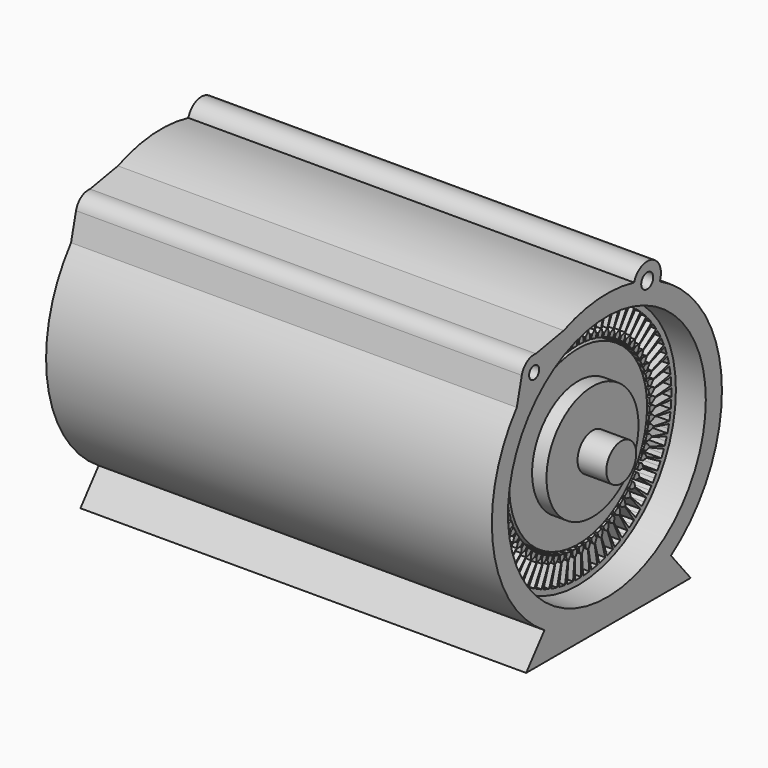
from build123d import *

# Parameters (mm, degrees)
F0_R            = 107.95
F0_R_2          = 78.74
F1_DEPTH        = 350.52
F3_DEPTH        = 350.52
F3_COPIES_COUNT = 72
F4_R            = 76.1265105647
F4_R_2          = 50.8
F5_DEPTH        = 350.52
F4_R_3          = 16.51
F6_DEPTH        = 368.3
F7_DEPTH        = 12.7
F8_DEPTH        = 38.1
F9_DEPTH        = 393.7
F10_R           = 109.22
F11_DEPTH       = 368.3
F12_DEPTH       = 25.4
F13_R           = 6.6206850407
F13_R_2         = 5.5641376478
F14_DEPTH       = 393.7


# Not quite as in the source:
# - a pattern or mirror of a feature is missing from the dataset's text; its kind, count and spacing are read off the source's solid


with BuildPart() as f1:
    # F0 (on Right) → F1 (new body)
    with BuildSketch(Plane.YZ):
        Circle(F0_R)
        Circle(F0_R_2, mode=Mode.SUBTRACT)
    extrude(amount=-F1_DEPTH)

    # F2 (on face) → F3 (cut)
    with BuildSketch(Plane.YZ):
        with BuildLine():
            ThreePointArc((0, 102.9899159424), (-1.6996566332, 102.9758901546), (-3.3988503274, 102.9338166118))
            Line((-3.3988503274, 102.9338166118), (-3.3988503274, 85.1252377033))
            Line((-3.3988503274, 85.1252377033), (-0.9682796663, 81.9411352277))
            Line((-0.9682796663, 81.9411352277), (-0.9682796663, 78.734046222))
            ThreePointArc((-0.9682796663, 78.734046222), (-0.4841489852, 78.7385115414), (0, 78.74))
            Line((0, 78.74), (0, 102.9899159424))
        make_face()
        with BuildLine():
            Line((3.3988503274, 85.1252377033), (3.3988503274, 102.9338166118))
            ThreePointArc((3.3988503274, 102.9338166118), (1.6996566332, 102.9758901546), (0, 102.9899159424))
            Line((0, 102.9899159424), (0, 78.74))
            ThreePointArc((0, 78.74), (0.4841489852, 78.7385115414), (0.9682796663, 78.734046222))
            Line((0.9682796663, 78.734046222), (0.9682796663, 81.9411352277))
            Line((0.9682796663, 81.9411352277), (3.3988503274, 85.1252377033))
        make_face()
    f3 = extrude(amount=-F3_DEPTH, mode=Mode.SUBTRACT)

    # F3_copies: F3 ×72 about axis
    f3_copies_axis = Axis((0, 0, 0), (1, 0, 0))
    for i in range(1, F3_COPIES_COUNT):
        add(f3.rotate(f3_copies_axis, i * 360 / F3_COPIES_COUNT), mode=Mode.SUBTRACT)


with BuildPart() as f5:
    # F4 (on Right) → F5 (new body)
    with BuildSketch(Plane.YZ):
        Circle(F4_R)
        Circle(F4_R_2, mode=Mode.SUBTRACT)
    extrude(amount=-F5_DEPTH)

    # F4 (on Right) → F6 (join)
    with BuildSketch(Plane.YZ):
        Circle(F4_R_2)
        Circle(F4_R_3, mode=Mode.SUBTRACT)
    extrude(amount=-F6_DEPTH)

    # F4 (on Right) → F7 (join)
    with BuildSketch(Plane.YZ):
        Circle(F4_R_2)
        Circle(F4_R_3, mode=Mode.SUBTRACT)
    extrude(amount=F7_DEPTH)


with BuildPart() as f8:
    # F4 (on Right) → F8 (new body)
    with BuildSketch(Plane.YZ):
        Circle(F4_R_3)
    extrude(amount=F8_DEPTH)


with BuildPart() as f9:
    # F4 (on Right) → F9 (new body)
    with BuildSketch(Plane.YZ):
        Circle(F4_R_3)
    extrude(amount=-F9_DEPTH)


with BuildPart() as f11:
    # F10 (on Right) → F11 (new body)
    with BuildSketch(Plane.YZ):
        with BuildLine():
            ThreePointArc((-90.6747852672, 88.9217820151), (-95.1978543213, 84.0616947999), (-99.4607591819, 78.9718771649))
            ThreePointArc((-99.4607591819, 78.9718771649), (-125.3190004758, -20.5948566332), (-68.9558634012, -106.6493736624))
            ThreePointArc((-68.9558634012, -106.6493736624), (1.0720603726, -126.9954750633), (70.74651636, -105.4700451452))
            ThreePointArc((70.74651636, -105.4700451452), (112.0575913933, -59.7670160803), (127, 0))
            ThreePointArc((127, 0), (108.4931230925, 66.0169844936), (58.3662639114, 112.793524801))
            ThreePointArc((58.3662639114, 112.793524801), (39.2223443362, 104.7597177346), (30.0618322387, 123.3907867))
            ThreePointArc((30.0618322387, 123.3907867), (-9.2649812179, 126.6615968754), (-47.6972368957, 117.7029039256))
            ThreePointArc((-47.6972368957, 117.7029039256), (-58.6459392445, 112.6483635484), (-69.0658774513, 106.5781617963))
            ThreePointArc((-69.0658774513, 106.5781617963), (-67.0706768882, 102.6747665417), (-66.3830520324, 98.3452755948))
            ThreePointArc((-66.3830520324, 98.3452755948), (-75.3028855949, 85.3175116386), (-90.6747852672, 88.9217820151))
        make_face()
        Circle(F10_R, mode=Mode.SUBTRACT)
        with BuildLine():
            ThreePointArc((-69.0658774513, 106.5781617963), (-80.3567468741, 98.3452755948), (-90.6747852672, 88.9217820151))
            ThreePointArc((-90.6747852672, 88.9217820151), (-75.3028855949, 85.3175116386), (-66.3830520324, 98.3452755948))
            ThreePointArc((-66.3830520324, 98.3452755948), (-67.0706768882, 102.6747665417), (-69.0658774513, 106.5781617963))
        make_face()
        with BuildLine():
            ThreePointArc((-93.9331000824, 101.6538676052), (-93.894176038, 94.8808623459), (-90.6747852672, 88.9217820151))
            ThreePointArc((-90.6747852672, 88.9217820151), (-80.3567468741, 98.3452755948), (-69.0658774513, 106.5781617963))
            ThreePointArc((-69.0658774513, 106.5781617963), (-73.1501559194, 110.3172927323), (-78.3660891177, 112.1764515833))
            ThreePointArc((-78.3660891177, 112.1764515833), (-88.1822358792, 109.9222298298), (-93.9331000824, 101.6538676052))
        make_face()
        with BuildLine():
            ThreePointArc((70.74651636, -105.4700451452), (1.0720603726, -126.9954750633), (-68.9558634012, -106.6493736624))
            Line((-68.9558634012, -106.6493736624), (-89.0998393297, -131.6837668419))
            Line((-89.0998393297, -131.6837668419), (92.5168767571, -131.6837668419))
            Line((92.5168767571, -131.6837668419), (70.74651636, -105.4700451452))
        make_face()
        with BuildLine():
            ThreePointArc((30.0618322387, 123.3907867), (44.5304113738, 118.9371366011), (58.3662639114, 112.793524801))
            ThreePointArc((58.3662639114, 112.793524801), (59.339683956, 115.7970367652), (59.6689311625, 118.9371366011))
            ThreePointArc((59.6689311625, 118.9371366011), (46.7822894612, 133.9072343454), (30.0618322387, 123.3907867))
        make_face()
        with BuildLine():
            ThreePointArc((30.0618322387, 123.3907867), (39.2223443362, 104.7597177346), (58.3662639114, 112.793524801))
            ThreePointArc((58.3662639114, 112.793524801), (44.5304113738, 118.9371366011), (30.0618322387, 123.3907867))
        make_face()
        with BuildLine():
            ThreePointArc((-78.3660891177, 112.1764515833), (-73.1501559194, 110.3172927323), (-69.0658774513, 106.5781617963))
            ThreePointArc((-69.0658774513, 106.5781617963), (-58.6459392445, 112.6483635484), (-47.6972368957, 117.7029039256))
            Line((-47.6972368957, 117.7029039256), (-78.3660891177, 112.1764515833))
        make_face()
        with BuildLine():
            Line((-93.9331000824, 101.6538676052), (-99.4607591819, 78.9718771649))
            ThreePointArc((-99.4607591819, 78.9718771649), (-95.1978543213, 84.0616947999), (-90.6747852672, 88.9217820151))
            ThreePointArc((-90.6747852672, 88.9217820151), (-93.894176038, 94.8808623459), (-93.9331000824, 101.6538676052))
        make_face()
    extrude(amount=-F11_DEPTH)

    # F12 (add): a face of the model
    f12_faces = [f11.faces().sort_by_distance(p)[0] for p in [
        (0, -8.9967932307, 122.9951977827),
    ]]
    extrude(f12_faces, amount=F12_DEPTH)

    # F13 (on face) → F14 (cut)
    with BuildSketch(Plane(origin=(-368.3, 0, 0), x_dir=(0, -1, 0), z_dir=(-1, 0, 0))):
        with Locations((-44.5304113738, 118.9371366011)):
            Circle(F13_R)
        with Locations((80.3567468741, 98.3452755948)):
            Circle(F13_R_2)
    extrude(amount=-F14_DEPTH, mode=Mode.SUBTRACT)


solid = Compound([f1.part, f5.part, f8.part, f9.part, f11.part])
